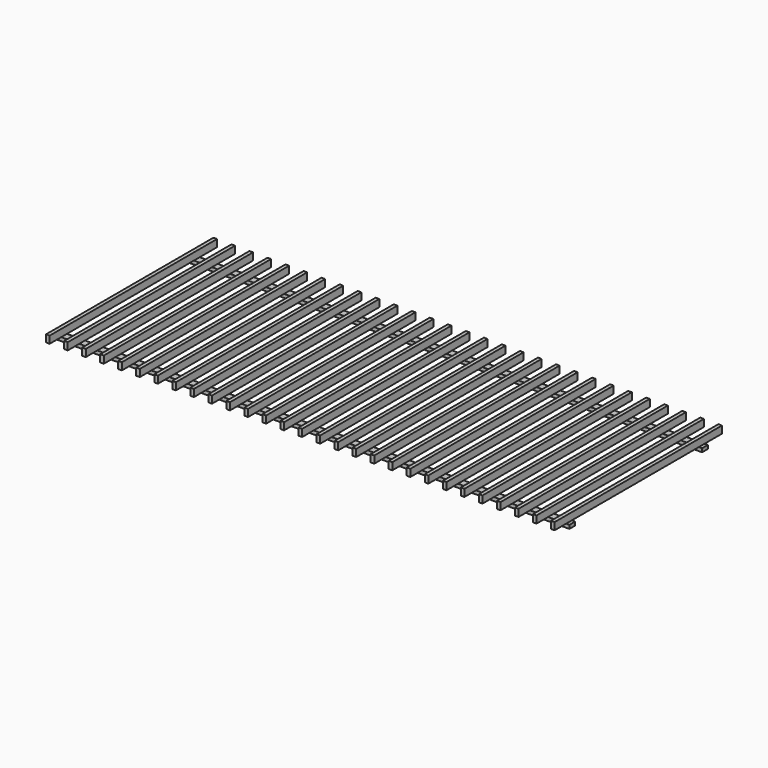
from build123d import *

# Parameters (mm, degrees)
F0_W     = 25
F0_H     = 1450
F1_DEPTH = 50
F2_W     = 3570
F2_H     = 50
F3_DEPTH = 25


# Not quite as in the source:
# - a feature names something its author has since deleted; it is built from what else it names


with BuildPart() as f1:
    # F0 (on Top) → F1 (new body)
    with BuildSketch(Plane.XY):
        with Locations((35, 775)):
            Rectangle(F0_W, F0_H)
    extrude(amount=F1_DEPTH)


with BuildPart() as f1b:
    # F0 (on Top) → F1, piece 2 (new body)
    with BuildSketch(Plane.XY):
        with Locations((160, 775)):
            Rectangle(F0_W, F0_H)
    extrude(amount=F1_DEPTH)


with BuildPart() as f1c:
    # F0 (on Top) → F1, piece 3 (new body)
    with BuildSketch(Plane.XY):
        with Locations((285, 775)):
            Rectangle(F0_W, F0_H)
    extrude(amount=F1_DEPTH)


with BuildPart() as f1d:
    # F0 (on Top) → F1, piece 4 (new body)
    with BuildSketch(Plane.XY):
        with Locations((410, 775)):
            Rectangle(F0_W, F0_H)
    extrude(amount=F1_DEPTH)


with BuildPart() as f1e:
    # F0 (on Top) → F1, piece 5 (new body)
    with BuildSketch(Plane.XY):
        with Locations((535, 775)):
            Rectangle(F0_W, F0_H)
    extrude(amount=F1_DEPTH)


with BuildPart() as f1f:
    # F0 (on Top) → F1, piece 6 (new body)
    with BuildSketch(Plane.XY):
        with Locations((660, 775)):
            Rectangle(F0_W, F0_H)
    extrude(amount=F1_DEPTH)


with BuildPart() as f1g:
    # F0 (on Top) → F1, piece 7 (new body)
    with BuildSketch(Plane.XY):
        with Locations((785, 775)):
            Rectangle(F0_W, F0_H)
    extrude(amount=F1_DEPTH)


with BuildPart() as f1h:
    # F0 (on Top) → F1, piece 8 (new body)
    with BuildSketch(Plane.XY):
        with Locations((910, 775)):
            Rectangle(F0_W, F0_H)
    extrude(amount=F1_DEPTH)


with BuildPart() as f1i:
    # F0 (on Top) → F1, piece 9 (new body)
    with BuildSketch(Plane.XY):
        with Locations((1035, 775)):
            Rectangle(F0_W, F0_H)
    extrude(amount=F1_DEPTH)


with BuildPart() as f1j:
    # F0 (on Top) → F1, piece 10 (new body)
    with BuildSketch(Plane.XY):
        with Locations((1160, 775)):
            Rectangle(F0_W, F0_H)
    extrude(amount=F1_DEPTH)


with BuildPart() as f1k:
    # F0 (on Top) → F1, piece 11 (new body)
    with BuildSketch(Plane.XY):
        with Locations((1285, 775)):
            Rectangle(F0_W, F0_H)
    extrude(amount=F1_DEPTH)


with BuildPart() as f1l:
    # F0 (on Top) → F1, piece 12 (new body)
    with BuildSketch(Plane.XY):
        with Locations((1410, 775)):
            Rectangle(F0_W, F0_H)
    extrude(amount=F1_DEPTH)


with BuildPart() as f1m:
    # F0 (on Top) → F1, piece 13 (new body)
    with BuildSketch(Plane.XY):
        with Locations((1535, 775)):
            Rectangle(F0_W, F0_H)
    extrude(amount=F1_DEPTH)


with BuildPart() as f1n:
    # F0 (on Top) → F1, piece 14 (new body)
    with BuildSketch(Plane.XY):
        with Locations((1660, 775)):
            Rectangle(F0_W, F0_H)
    extrude(amount=F1_DEPTH)


with BuildPart() as f1o:
    # F0 (on Top) → F1, piece 15 (new body)
    with BuildSketch(Plane.XY):
        with Locations((1785, 775)):
            Rectangle(F0_W, F0_H)
    extrude(amount=F1_DEPTH)


with BuildPart() as f1p:
    # F0 (on Top) → F1, piece 16 (new body)
    with BuildSketch(Plane.XY):
        with Locations((1910, 775)):
            Rectangle(F0_W, F0_H)
    extrude(amount=F1_DEPTH)


with BuildPart() as f1q:
    # F0 (on Top) → F1, piece 17 (new body)
    with BuildSketch(Plane.XY):
        with Locations((2035, 775)):
            Rectangle(F0_W, F0_H)
    extrude(amount=F1_DEPTH)


with BuildPart() as f1r:
    # F0 (on Top) → F1, piece 18 (new body)
    with BuildSketch(Plane.XY):
        with Locations((2160, 775)):
            Rectangle(F0_W, F0_H)
    extrude(amount=F1_DEPTH)


with BuildPart() as f1s:
    # F0 (on Top) → F1, piece 19 (new body)
    with BuildSketch(Plane.XY):
        with Locations((2285, 775)):
            Rectangle(F0_W, F0_H)
    extrude(amount=F1_DEPTH)


with BuildPart() as f1t:
    # F0 (on Top) → F1, piece 20 (new body)
    with BuildSketch(Plane.XY):
        with Locations((2410, 775)):
            Rectangle(F0_W, F0_H)
    extrude(amount=F1_DEPTH)


with BuildPart() as f1u:
    # F0 (on Top) → F1, piece 21 (new body)
    with BuildSketch(Plane.XY):
        with Locations((2535, 775)):
            Rectangle(F0_W, F0_H)
    extrude(amount=F1_DEPTH)


with BuildPart() as f1v:
    # F0 (on Top) → F1, piece 22 (new body)
    with BuildSketch(Plane.XY):
        with Locations((2660, 775)):
            Rectangle(F0_W, F0_H)
    extrude(amount=F1_DEPTH)


with BuildPart() as f1w:
    # F0 (on Top) → F1, piece 23 (new body)
    with BuildSketch(Plane.XY):
        with Locations((2785, 775)):
            Rectangle(F0_W, F0_H)
    extrude(amount=F1_DEPTH)


with BuildPart() as f1x:
    # F0 (on Top) → F1, piece 24 (new body)
    with BuildSketch(Plane.XY):
        with Locations((2910, 775)):
            Rectangle(F0_W, F0_H)
    extrude(amount=F1_DEPTH)


with BuildPart() as f1y:
    # F0 (on Top) → F1, piece 25 (new body)
    with BuildSketch(Plane.XY):
        with Locations((3035, 775)):
            Rectangle(F0_W, F0_H)
    extrude(amount=F1_DEPTH)


with BuildPart() as f1z:
    # F0 (on Top) → F1, piece 26 (new body)
    with BuildSketch(Plane.XY):
        with Locations((3160, 775)):
            Rectangle(F0_W, F0_H)
    extrude(amount=F1_DEPTH)


with BuildPart() as f1ba:
    # F0 (on Top) → F1, piece 27 (new body)
    with BuildSketch(Plane.XY):
        with Locations((3285, 775)):
            Rectangle(F0_W, F0_H)
    extrude(amount=F1_DEPTH)


with BuildPart() as f1bb:
    # F0 (on Top) → F1, piece 28 (new body)
    with BuildSketch(Plane.XY):
        with Locations((3410, 775)):
            Rectangle(F0_W, F0_H)
    extrude(amount=F1_DEPTH)


with BuildPart() as f1bc:
    # F0 (on Top) → F1, piece 29 (new body)
    with BuildSketch(Plane.XY):
        with Locations((3535, 775)):
            Rectangle(F0_W, F0_H)
    extrude(amount=F1_DEPTH)


with BuildPart() as f3:
    # F2 (on Top) → F3 (new body)
    with BuildSketch(Plane.XY):
        with Locations((1785, 175)):
            Rectangle(F2_W, F2_H)
    extrude(amount=-F3_DEPTH)


with BuildPart() as f3b:
    # F2 (on Top) → F3, piece 2 (new body)
    with BuildSketch(Plane.XY):
        with Locations((1785, 1325)):
            Rectangle(F2_W, F2_H)
    extrude(amount=-F3_DEPTH)


solid = Compound([f1.part, f1b.part, f1c.part, f1d.part, f1e.part, f1f.part, f1g.part, f1h.part, f1i.part, f1j.part, f1k.part, f1l.part, f1m.part, f1n.part, f1o.part, f1p.part, f1q.part, f1r.part, f1s.part, f1t.part, f1u.part, f1v.part, f1w.part, f1x.part, f1y.part, f1z.part, f1ba.part, f1bb.part, f1bc.part, f3.part, f3b.part])
